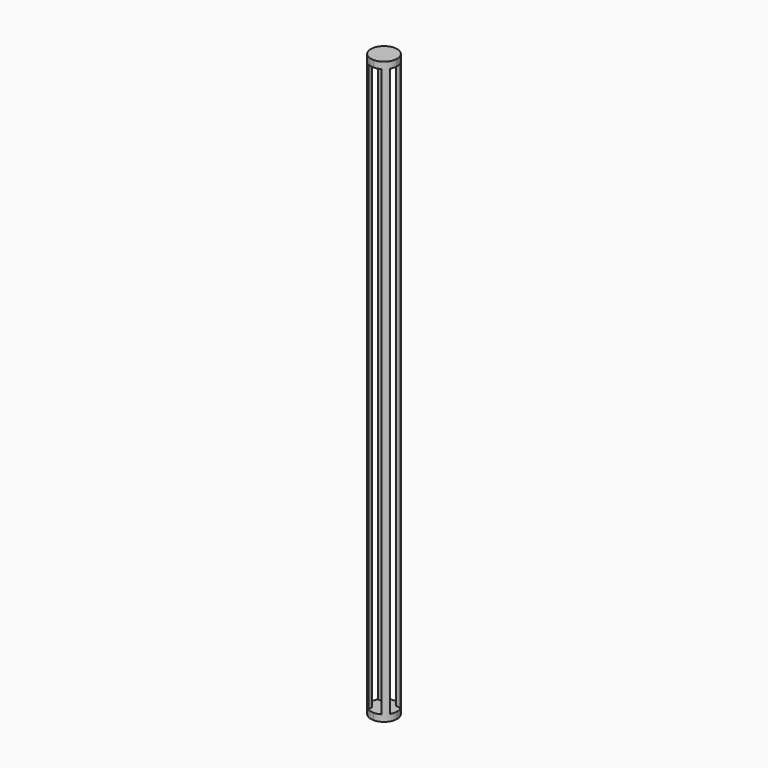
from build123d import *

# Parameters (mm, degrees)
F0_W          = 5.08
F0_H          = 5.08
F1_DEPTH      = 36.83
F1_DEPTH_BACK = 75.184
F2_W          = 2.54
F2_H          = 109.474
F3_DEPTH      = 23.114
F4_W          = 2.54
F4_H          = 109.474
F5_DEPTH      = 4.5777483376
F5_DEPTH_BACK = 29.972
F6_T1_DEPTH   = 124.714


# Not quite as in the source:
# - a fillet or chamfer that OpenCascade refuses, or shapes differently, is made with other operations: its cross-section is extruded or revolved along the edge and cut away or added


with BuildPart() as f1:
    # F0 (on Top) → F1 (new body, two sides)
    with BuildSketch(Plane.XY) as f1_sk:
        with Locations((-2.0367483376, -3.0882195887)):
            Rectangle(F0_W, F0_H)
    extrude(amount=F1_DEPTH)
    extrude(f1_sk.sketch, amount=-F1_DEPTH_BACK)

    # F2 (on Front) → F3 (cut)
    with BuildSketch(Plane.XZ):
        with Locations((-2.0367483376, -19.177)):
            Rectangle(F2_W, F2_H)
    extrude(amount=F3_DEPTH, mode=Mode.SUBTRACT)

    # F4 (on Right) → F5 (cut, two sides)
    with BuildSketch(Plane.YZ) as f5_sk:
        with Locations((-3.0882195887, -19.177)):
            Rectangle(F4_W, F4_H)
    extrude(amount=-F5_DEPTH, mode=Mode.SUBTRACT)
    extrude(f5_sk.sketch, amount=F5_DEPTH_BACK, mode=Mode.SUBTRACT)

    # F6: fillet of radius 2.54 on 4 edges, made by hand

    # F6_s2 → F6_t1 (cut)
    with BuildSketch(Plane.XY.offset(-81.534)):
        with BuildLine():
            ThreePointArc((0.5032516624, -3.0882195887), (-0.2406971133, -4.8842708129), (-2.0367483376, -5.6282195887))
            Line((-2.0367483376, -5.6282195887), (0.5032516624, -5.6282195887))
            Line((0.5032516624, -5.6282195887), (0.5032516624, -3.0882195887))
        make_face()
        with BuildLine():
            ThreePointArc((-4.5767483376, -3.0882195887), (-3.8327995618, -4.8842708129), (-2.0367483376, -5.6282195887))
            Line((-2.0367483376, -5.6282195887), (-4.5767483376, -5.6282195887))
            Line((-4.5767483376, -5.6282195887), (-4.5767483376, -3.0882195887))
        make_face()
        with BuildLine():
            ThreePointArc((-2.0367483376, -0.5482195887), (-3.8327995618, -1.2921683645), (-4.5767483376, -3.0882195887))
            Line((-4.5767483376, -3.0882195887), (-4.5767483376, -0.5482195887))
            Line((-4.5767483376, -0.5482195887), (-2.0367483376, -0.5482195887))
        make_face()
        with BuildLine():
            ThreePointArc((-2.0367483376, -0.5482195887), (-0.2406971133, -1.2921683645), (0.5032516624, -3.0882195887))
            Line((0.5032516624, -3.0882195887), (0.5032516624, -0.5482195887))
            Line((0.5032516624, -0.5482195887), (-2.0367483376, -0.5482195887))
        make_face()
    extrude(amount=F6_T1_DEPTH, mode=Mode.SUBTRACT)


solid = f1.part
